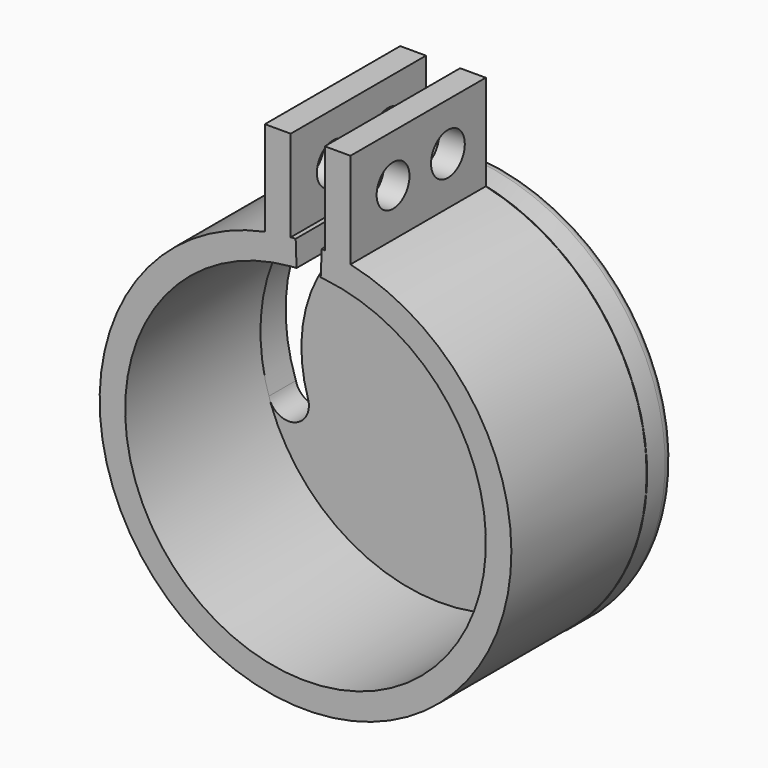
from build123d import *

# Parameters (mm, degrees)
F1_DEPTH = 15
F3_DEPTH = 3
F4_R     = 1
F5_R     = 1.821901794
F5_R_2   = 1.8725831309
F6_DEPTH = 25


with BuildPart() as f1:
    # F0 (on Front) → F1 (new body)
    with BuildSketch(Plane.XZ):
        with BuildLine():
            ThreePointArc((-1.3153538917, 15.9458409668), (-1.0543071799, 15.9652258478), (-0.7929782714, 15.9803374639))
            Line((-0.7929782714, 15.9803374639), (-0.8730364945, 18.2393764119))
            ThreePointArc((-0.8730364945, 18.2393764119), (-1.0942757438, 18.2274409946), (-1.3153538917, 18.2128220975))
            Line((-1.3153538917, 18.2128220975), (-1.3153538917, 15.9458409668))
        make_face()
        with BuildLine():
            ThreePointArc((1.710430308, 15.9083131778), (-0.1984273858, -15.9987695331), (-1.3153538917, 15.9458409668))
            Line((-1.3153538917, 15.9458409668), (-3.6037638783, 15.9458409668))
            Line((-3.6037638783, 15.9458409668), (-3.6037638783, 17.901115343))
            ThreePointArc((-3.6037638783, 17.901115343), (-0.1952417623, -18.2592148043), (3.9857214978, 17.8199626475))
            Line((3.9857214978, 17.8199626475), (3.9857214978, 15.9083131778))
            Line((3.9857214978, 15.9083131778), (1.710430308, 15.9083131778))
        make_face()
        with BuildLine():
            Line((-3.6037638783, 15.9458409668), (-1.3153538917, 15.9458409668))
            Line((-1.3153538917, 15.9458409668), (-1.3153538917, 18.2128220975))
            ThreePointArc((-1.3153538917, 18.2128220975), (-2.4644918714, 18.0931844746), (-3.6037638783, 17.901115343))
            Line((-3.6037638783, 17.901115343), (-3.6037638783, 15.9458409668))
        make_face()
        with BuildLine():
            Line((1.710430308, 18.1799744988), (1.710430308, 15.9083131778))
            Line((1.710430308, 15.9083131778), (3.9857214978, 15.9083131778))
            Line((3.9857214978, 15.9083131778), (3.9857214978, 17.8199626475))
            ThreePointArc((3.9857214978, 17.8199626475), (2.8537586587, 18.0358838467), (1.710430308, 18.1799744988))
        make_face()
        with BuildLine():
            ThreePointArc((1.3463109011, 15.9432571), (1.5284704689, 15.926825736), (1.710430308, 15.9083131778))
            Line((1.710430308, 15.9083131778), (1.710430308, 18.1799744988))
            ThreePointArc((1.710430308, 18.1799744988), (1.5756035958, 18.1921553952), (1.4406902841, 18.2033364008))
            Line((1.4406902841, 18.2033364008), (1.3463109011, 15.9432571))
        make_face()
        with BuildLine():
            ThreePointArc((-3.6037638783, 17.901115343), (-2.4644918714, 18.0931844746), (-1.3153538917, 18.2128220975))
            Line((-1.3153538917, 18.2128220975), (-1.3153538917, 26.3016127771))
            Line((-1.3153538917, 26.3016127771), (-3.6037638783, 26.3016127771))
            Line((-3.6037638783, 26.3016127771), (-3.6037638783, 17.901115343))
        make_face()
        with BuildLine():
            Line((1.710430308, 26.3016127771), (1.710430308, 18.1799744988))
            ThreePointArc((1.710430308, 18.1799744988), (2.8537586587, 18.0358838467), (3.9857214978, 17.8199626475))
            Line((3.9857214978, 17.8199626475), (3.9857214978, 26.3016127771))
            Line((3.9857214978, 26.3016127771), (1.710430308, 26.3016127771))
        make_face()
    extrude(amount=F1_DEPTH)

    # F5 (on face) → F6 (cut)
    with BuildSketch(Plane.YZ.offset(3.9857214978)):
        with Locations((-10.2766146883, 22.0607877123)):
            Circle(F5_R)
        with Locations((-4.1950447485, 22.0607877123)):
            Circle(F5_R_2)
    extrude(amount=-F6_DEPTH, mode=Mode.SUBTRACT)


with BuildPart() as f3:
    # F2 (on face) → F3 (new body)
    with BuildSketch(Plane(origin=(0, 0, 0), x_dir=(-1, 0, 0), z_dir=(0, 1, 0))):
        with BuildLine():
            ThreePointArc((15.254548473, -4.8268779645), (13.0876587907, -6.1644776131), (11.7500591421, -3.9975879308))
            ThreePointArc((11.7500591421, -3.9975879308), (0.5173215514, 12.7592430058), (-13.2079693725, -2.0252815342))
            ThreePointArc((-13.2079693725, -2.0252815342), (-14.5396358049, -3.2329563244), (-15.8713022373, -2.0252815342))
            ThreePointArc((-15.8713022373, -2.0252815342), (-12.7555816036, 10.3110617982), (-1.3463109011, 15.9432571))
            Line((-1.3463109011, 15.9432571), (-1.4583122663, 18.2436864304))
            ThreePointArc((-1.4583122663, 18.2436864304), (0.2273298413, -18.3004669443), (1.0046831878, 18.2742819538))
            Line((1.0046831878, 18.2742819538), (0.7929782714, 15.9803374639))
            ThreePointArc((0.7929782714, 15.9803374639), (13.3814969398, 9.3004976117), (15.254548473, -4.8268779645))
        make_face()
    extrude(amount=F3_DEPTH)

    # F4
    f4_edges = [f3.edges().sort_by_distance(p)[0] for p in [
        (-0.22733, 3, -18.300467),
    ]]
    fillet(f4_edges, radius=F4_R)


solid = Compound([f1.part, f3.part])
